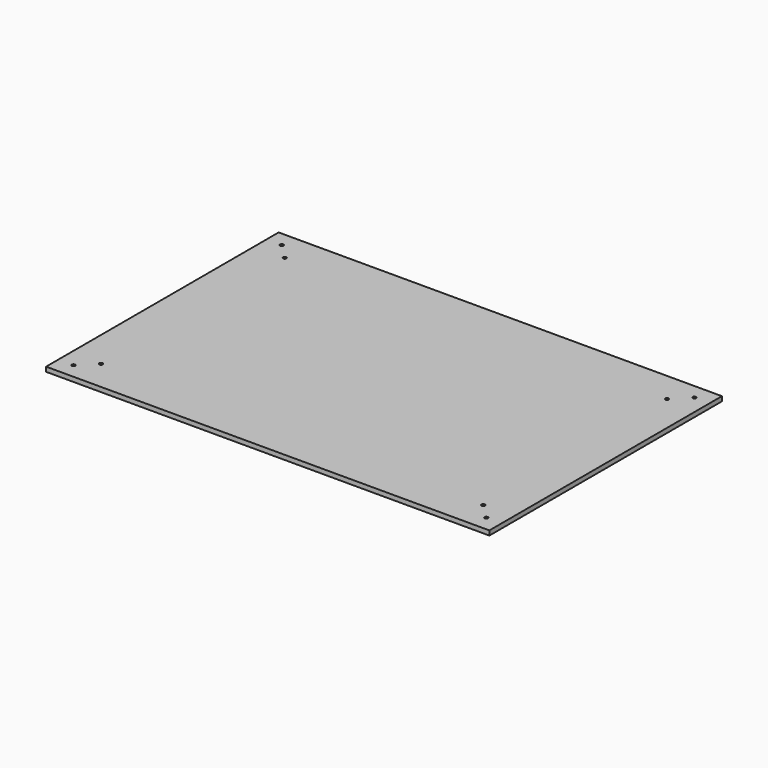
from build123d import *

# Parameters (mm, degrees)
F0_W             = 581
F0_H             = 381
F1_DEPTH         = 6
F2_D             = 4.5
F2_COPIES2_COUNT = 2
F2_COPIES2_PITCH = 611.949344


# Not quite as in the source:
# - a pattern or mirror of a feature is missing from the dataset's text; its kind, count and spacing are read off the source's solid


with BuildPart() as f1:
    # F0 (on Top) → F1 (new body)
    with BuildSketch(Plane.XY):
        Rectangle(F0_W, F0_H)
    extrude(amount=F1_DEPTH)

    # F2 (through all)
    with Locations(Plane(origin=(0, 0, 0), x_dir=(1, 0, 0), z_dir=(0, 0, -1))):
        with Locations((-250.5, -150.5), (-270.5, -170.5)):
            f2 = Hole(F2_D / 2)

    # F2_copies: F2 across plane
    add(f2.mirror(Plane(origin=(0, 0, 0), x_dir=(0, 0, 1), z_dir=(1, 0, 0))), mode=Mode.SUBTRACT)

    # F2_copies1: F2 across plane
    add(f2.mirror(Plane(origin=(0, 0, 0), x_dir=(0, 0, -1), z_dir=(0, -1, 0))), mode=Mode.SUBTRACT)

    # F2_copies2: F2 ×2
    with Locations(*[Vector(0.8513776587, -0.5245532216, 0) * (i * F2_COPIES2_PITCH) for i in range(1, F2_COPIES2_COUNT)]):
        add(f2, mode=Mode.SUBTRACT)


solid = f1.part
